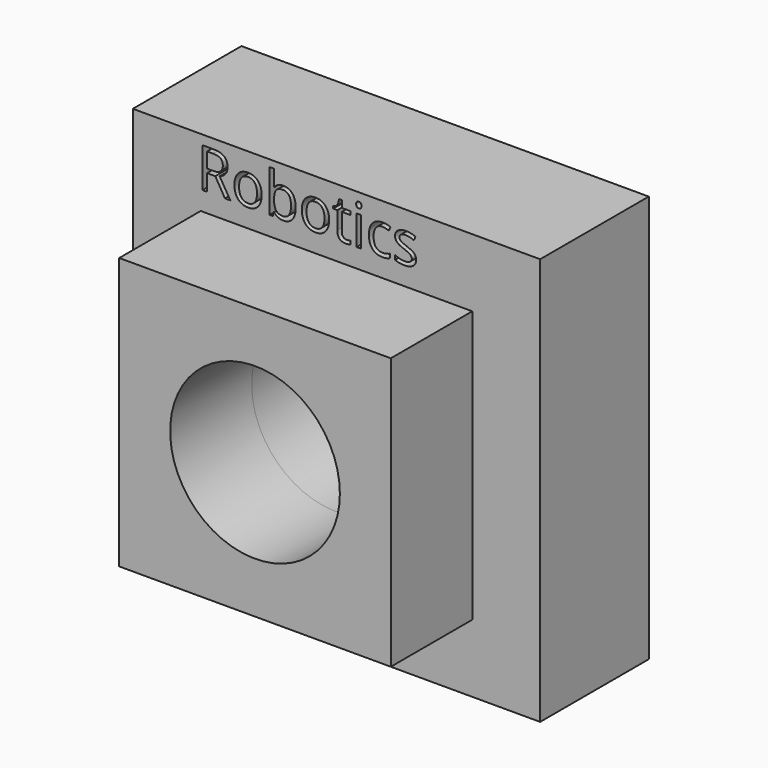
from build123d import *

# Parameters (mm, degrees)
F0_W         = 101.6
F0_H         = 101.6
F0_R         = 31.75
F1_DEPTH     = 38.1
F0_W_2       = 152.4
F0_H_2       = 152.4
F2_DEPTH     = 50.8
F3_TEXT_SIZE = 20.739927681
F4_DEPTH     = 88.901


# Not quite as in the source:
# - Text() gives the source's letters only with a copy of the font that has no kerning and outlines rounded to 1/6400 em; it was checked with that copy


with BuildPart() as f1:
    # F0 (on Front) → F1 (new body)
    with BuildSketch(Plane.XZ):
        Rectangle(F0_W, F0_H)
        Circle(F0_R, mode=Mode.SUBTRACT)
    extrude(amount=F1_DEPTH)


with BuildPart() as f2:
    # F0 (on Front) → F2 (new body)
    with BuildSketch(Plane.XZ):
        Rectangle(F0_W_2, F0_H_2)
        Rectangle(F0_W, F0_H, mode=Mode.SUBTRACT)
        Rectangle(F0_W, F0_H)
        Circle(F0_R, mode=Mode.SUBTRACT)
    extrude(amount=-F2_DEPTH)

    # F3 (on face) → F4 (cut, through all)
    with BuildSketch(Plane.XZ.offset(38.1)):
        with Locations((-52.1724186838, 57.887416333)):
            Text('Robotics', F3_TEXT_SIZE, font='Open Sans', text_align=(TextAlign.LEFT, TextAlign.BOTTOM))
    extrude(amount=-F4_DEPTH, mode=Mode.SUBTRACT)


solid = Compound([f1.part, f2.part])
